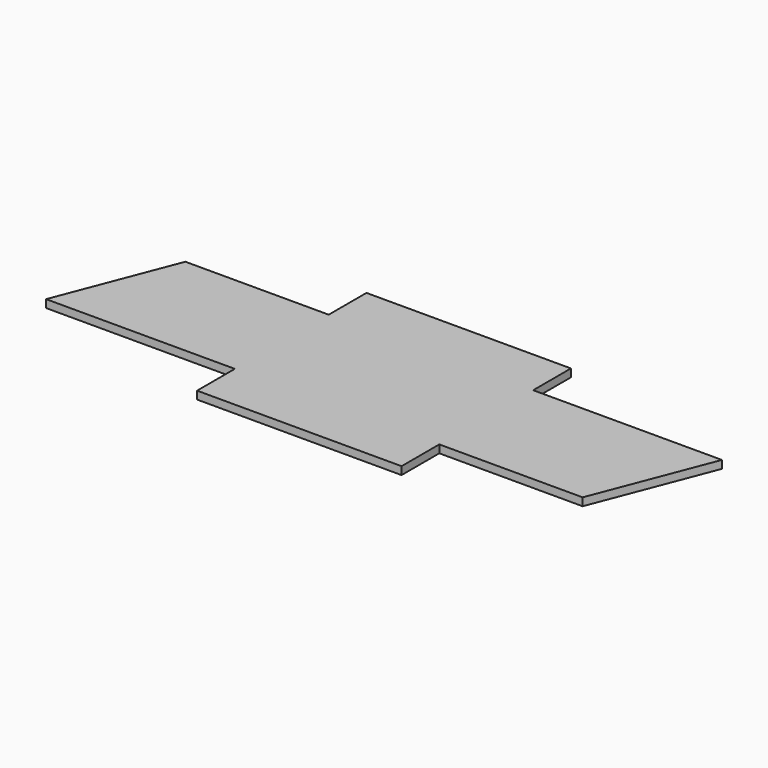
from build123d import *

# Parameters (mm, degrees)
F1_DEPTH = 3.175


# Not quite as in the source:
# - the program builds the solid bodies; features that only make, move or delete a surface that nothing else refers to are left out


with BuildPart() as f1:
    # F0 (on Top) → F1 (new body)
    with BuildSketch(Plane.XY):
        Polygon((82.55, 0), (0, 0), (0, -19.05), (-57.8740507578, -19.05), (-76.2, -66.4293159973), (0, -66.4293159973), (0, -85.4793159973), (82.55, -85.4793159973), (82.55, -66.4293159973), (140.4240507578, -66.4293159973), (158.75, -19.05), (82.55, -19.05), align=None)
    extrude(amount=F1_DEPTH)


solid = f1.part
